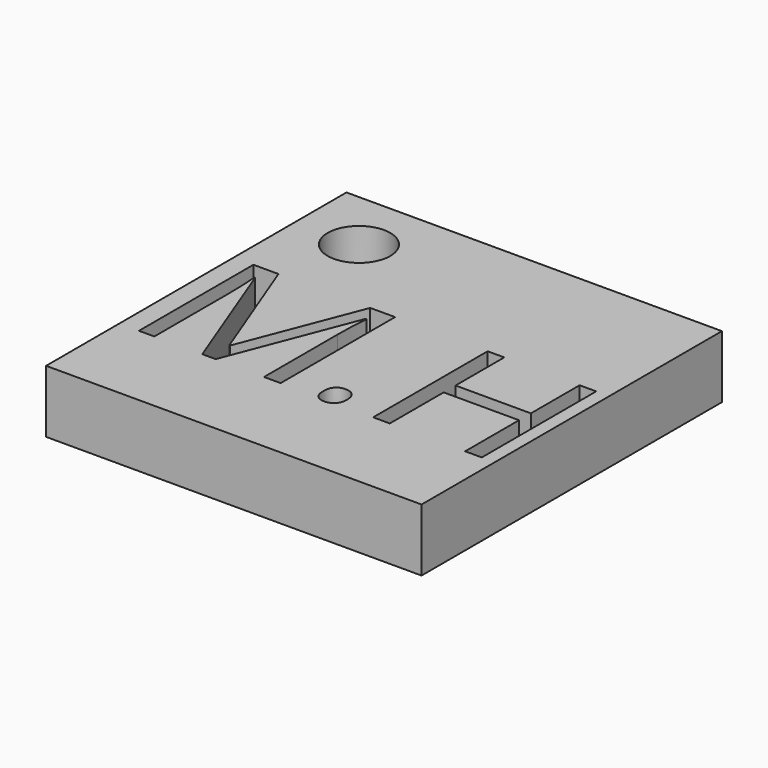
from build123d import *

# Parameters (mm, degrees)
F0_W         = 30
F0_H         = 30
F0_R         = 2.5
F1_DEPTH     = 5
F2_TEXT_SIZE = 16.009338781
F3_DEPTH     = 25


# Not quite as in the source:
# - Text() gives the source's letters only with a copy of the font that has no kerning and outlines rounded to 1/6400 em; it was checked with that copy


with BuildPart() as f1:
    # F0 (on Top) → F1 (new body)
    with BuildSketch(Plane.XY):
        with Locations((15, 15)):
            Rectangle(F0_W, F0_H)
        with Locations((5, 25)):
            Circle(F0_R, mode=Mode.SUBTRACT)
    extrude(amount=F1_DEPTH)

    # F2 (on face) → F3 (cut)
    with BuildSketch(Plane.XY.offset(5)):
        with Locations((0, 7.3130383563)):
            Text('M.H', F2_TEXT_SIZE, font='Open Sans', text_align=(TextAlign.LEFT, TextAlign.BOTTOM))
    extrude(amount=-F3_DEPTH, mode=Mode.SUBTRACT)


solid = f1.part
